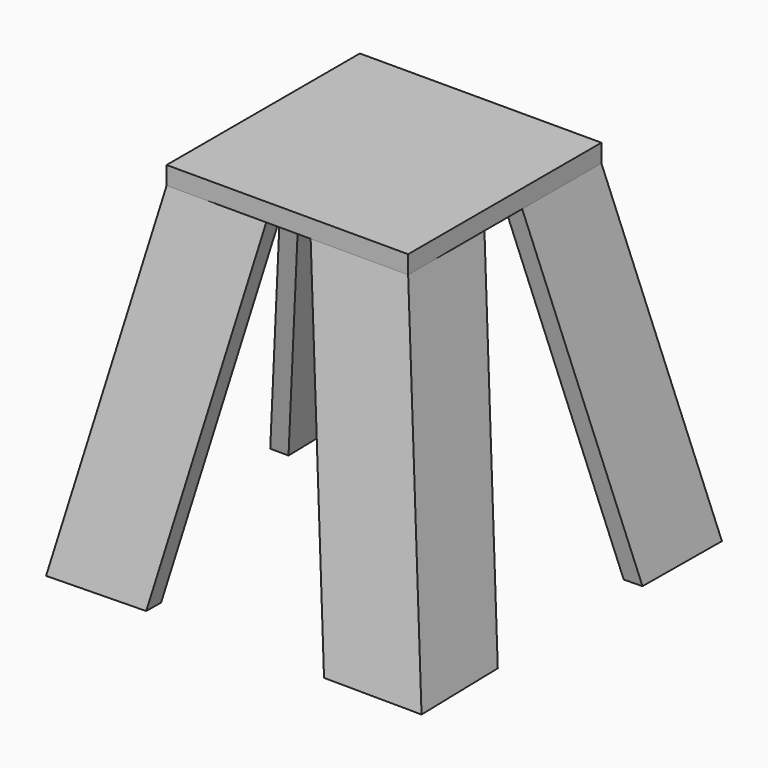
from build123d import *

# Parameters (mm, degrees)
F0_W           = 127
F0_H           = 127
F1_DEPTH       = 4.7625
F10_COUNT      = 4
F11_W          = 256.6241295266
F11_H          = 47.3635128975
F11_W_2        = 208.3994597018
F11_H_2        = 50.8081313799
F12_DEPTH      = 101.757131785
F12_DEPTH_BACK = 101.757131785
F13_W          = 127
F13_H          = 127
F14_DEPTH      = 9.525


# Not quite as in the source:
# - a length typed as a fraction of an inch, garbled in the dataset ("3 / 203.2 mm" for 3/8 in), is restored


with BuildPart() as f1:
    # F0 (on Top) → F1 (new body, symmetric)
    with BuildSketch(Plane.XY):
        Rectangle(F0_W, F0_H)
    extrude(amount=F1_DEPTH, both=True)

    # F8: sweep along a path in F7
    with BuildLine(Plane(origin=(0, 0, 0), x_dir=(-0.7071067812, 0.7071067812, 0), z_dir=(0.7071067812, 0.7071067812, 0))) as f8_path:
        Line((-80.7717935616, 27.4836799613), (-142.8134914441, -194.0487337554))
    # F6 (on offset) → F8 (sweep)
    with BuildSketch(Plane(origin=(26.5098868769, -26.5098868769, -212.6199938753), x_dir=(0.9924329475, 0.015191802, 0.1218443842), z_dir=(0.122787804, -0.122787804, -0.984807753))):
        Polygon((75.0423507795, 76.2), (24.2423507795, 76.2), (24.2423507795, 66.675), (65.5173507795, 66.675), (65.5173507795, 25.4), (75.0423507795, 25.4), align=None)
    sweep(path=f8_path.line)


with BuildPart() as f10_1:
    # F10: instance of F1
    add(f1.part.rotate(Axis((0, 0, -49.5498217642), (0, 0, -1)), 1 * 360 / F10_COUNT))


with BuildPart() as f10_2:
    # F10: instance of F1
    add(f1.part.rotate(Axis((0, 0, -49.5498217642), (0, 0, -1)), 2 * 360 / F10_COUNT))


with BuildPart() as f10_3:
    # F10: instance of F1
    add(f1.part.rotate(Axis((0, 0, -49.5498217642), (0, 0, -1)), 3 * 360 / F10_COUNT))


with BuildPart() as f12_tool:
    # F11 (on Front) → F12 (new body, two sides)
    with BuildSketch(Plane.XZ) as f12_sk:
        with Locations((2.9296859242, -206.2442564488)):
            Rectangle(F11_W, F11_H)
        with Locations((-6.5430181316, 20.6415656899)):
            Rectangle(F11_W_2, F11_H_2)
    extrude(amount=-F12_DEPTH)
    extrude(f12_sk.sketch, amount=F12_DEPTH_BACK)


with BuildPart() as f1_1:
    add(f1.part)

    # F12: cut by f12_tool
    add(f12_tool.part, mode=Mode.SUBTRACT)



with BuildPart() as f10_1_1:
    add(f10_1.part)

    # F12: cut by f12_tool
    add(f12_tool.part, mode=Mode.SUBTRACT)


with BuildPart() as f10_2_1:
    add(f10_2.part)

    # F12: cut by f12_tool
    add(f12_tool.part, mode=Mode.SUBTRACT)


with BuildPart() as f10_3_1:
    add(f10_3.part)

    # F12: cut by f12_tool
    add(f12_tool.part, mode=Mode.SUBTRACT)


with BuildPart() as f1_2:
    add(f1_1.part)

    add(f10_1_1.part)  # F14 merges F10_1

    add(f10_2_1.part)  # F14 merges F10_2

    add(f10_3_1.part)  # F14 merges F10_3
    # F13 (on face) → F14 (join)
    with BuildSketch(Plane.XY.offset(-4.7625)):
        Rectangle(F13_W, F13_H)
    extrude(amount=F14_DEPTH)


solid = f1_2.part
